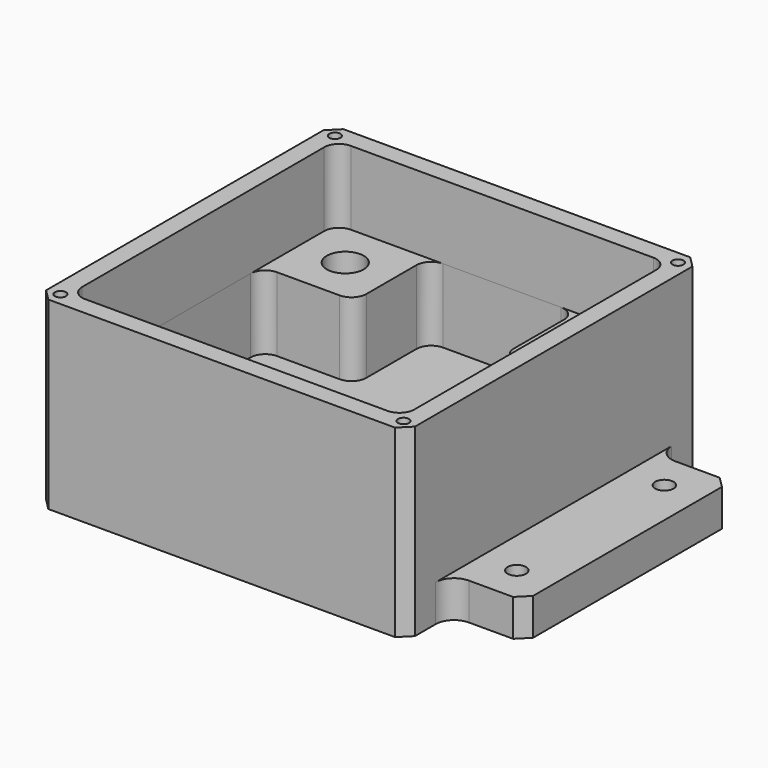
from build123d import *

# Parameters (mm, degrees)
F1_DEPTH     = 50
F2_W         = 20
F2_H         = 100
F3_DEPTH     = 40
F4_R         = 2.5
F5_DEPTH     = 10
F6_W         = 90
F6_H         = 90
F7_DEPTH     = 20
F8_R         = 5
F9_DEPTH     = 20
F10_R        = 1.5
F11_DEPTH    = 40
F12_SIZE     = 3
F13_T1_DEPTH = 30
F13_T3_DEPTH = 30
F13_T5_DEPTH = 30


# Not quite as in the source:
# - a fillet or chamfer that OpenCascade refuses, or shapes differently, is made with other operations: its cross-section is extruded or revolved along the edge and cut away or added


with BuildPart() as f1:
    # F0 (on Top) → F1 (new body)
    with BuildSketch(Plane.XY):
        Polygon((-50, -50), (50, -50), (70, -50), (70, 50), (50, 50), (-50, 50), align=None)
    extrude(amount=F1_DEPTH)

    # F2 (on face) → F3 (cut)
    with BuildSketch(Plane.XY.offset(50)):
        with Locations((60, 0)):
            Rectangle(F2_W, F2_H)
    extrude(amount=-F3_DEPTH, mode=Mode.SUBTRACT)

    # F4 (on face) → F5 (cut, through all)
    with BuildSketch(Plane.XY.offset(10)):
        with BuildLine():
            Line((50, -40), (50, -50))
            Line((50, -50), (70, -50))
            Line((70, -50), (70, -35))
            Line((70, -35), (55, -35))
            ThreePointArc((55, -35), (51.4644660941, -36.4644660941), (50, -40))
        make_face()
        with Locations((60, -25)):
            Circle(F4_R)
        with Locations((60, 25)):
            Circle(F4_R)
        with BuildLine():
            ThreePointArc((50, 40), (51.4644660941, 36.4644660941), (55, 35))
            Line((55, 35), (70, 35))
            Line((70, 35), (70, 50))
            Line((70, 50), (50, 50))
            Line((50, 50), (50, 40))
        make_face()
    extrude(amount=-F5_DEPTH, mode=Mode.SUBTRACT)

    # F6 (on face) → F7 (cut)
    with BuildSketch(Plane.XY.offset(50)):
        Rectangle(F6_W, F6_H)
    extrude(amount=-F7_DEPTH, mode=Mode.SUBTRACT)

    # F8 (on face) → F9 (cut)
    with BuildSketch(Plane.XY.offset(30)):
        with Locations((-32.5000025332, 32.5000174344)):
            Circle(F8_R)
        Polygon((-45.0000017881, 20.0000017881), (-45.0000017881, -20.0000017881), (-20.0000017881, -20.0000017881), (-20.0000017881, -45.0000017881), (20.0000017881, -45.0000017881), (20.0000017881, -20.0000017881), (45.0000017881, -20.0000017881), (45.0000017881, 20.0000017881), (20.0000017881, 20.0000017881), (20.0000017881, 45.0000017881), (-20.0000017881, 45.0000017881), (-20.0000017881, 20.0000017881), align=None)
        with Locations((-32.5000025332, -32.5000174344)):
            Circle(F8_R)
        with Locations((32.5000025332, 32.5000174344)):
            Circle(F8_R)
        with Locations((32.5000025332, -32.5000174344)):
            Circle(F8_R)
    extrude(amount=-F9_DEPTH, mode=Mode.SUBTRACT)

    # F10 (on face) → F11 (cut)
    with BuildSketch(Plane.XY.offset(50)):
        with Locations((-46.5, 46.5)):
            Circle(F10_R)
        with Locations((-46.5, -46.5)):
            Circle(F10_R)
        with Locations((46.5, 46.5)):
            Circle(F10_R)
        with Locations((46.5, -46.5)):
            Circle(F10_R)
    extrude(amount=-F11_DEPTH, mode=Mode.SUBTRACT)

    # F12
    f12_edges = [f1.edges().sort_by_distance(p)[0] for p in [
        (70, -35, 5),
        (70, 35, 5),
        (50, -50, 25),
        (-50, -50, 25),
        (50, 50, 25),
        (-50, 50, 25),
    ]]
    chamfer(f12_edges, length=F12_SIZE)

    # F13: fillet of radius 4 on 16 edges, made by hand

    # F13_s2 → F13_t1 (join)
    with BuildSketch(Plane.XY.offset(20)):
        with BuildLine():
            ThreePointArc((-45, 41), (-43.8284271247, 43.8284271247), (-41, 45))
            Line((-41, 45), (-45, 45))
            Line((-45, 45), (-45, 41))
        make_face()
        with BuildLine():
            ThreePointArc((45, 41), (43.8284271247, 43.8284271247), (41, 45))
            Line((41, 45), (45, 45))
            Line((45, 45), (45, 41))
        make_face()
        with BuildLine():
            ThreePointArc((41, -45), (43.8284271247, -43.8284271247), (45, -41))
            Line((45, -41), (45, -45))
            Line((45, -45), (41, -45))
        make_face()
        with BuildLine():
            ThreePointArc((-41, -45), (-43.8284271247, -43.8284271247), (-45, -41))
            Line((-45, -41), (-45, -45))
            Line((-45, -45), (-41, -45))
        make_face()
    extrude(amount=F13_T1_DEPTH)

    # F13_s4 → F13_t3 (join)
    with BuildSketch(Plane.XY):
        with BuildLine():
            ThreePointArc((-41.0000017881, 20.0000017881), (-43.8284289129, 18.8284289129), (-45.0000017881, 16.0000017881))
            Line((-45.0000017881, 16.0000017881), (-45.0000017881, 20.0000017881))
            Line((-45.0000017881, 20.0000017881), (-41.0000017881, 20.0000017881))
        make_face()
        with BuildLine():
            ThreePointArc((-20.0000017881, 41.0000017881), (-18.8284289129, 43.8284289129), (-16.0000017881, 45.0000017881))
            Line((-16.0000017881, 45.0000017881), (-20.0000017881, 45.0000017881))
            Line((-20.0000017881, 45.0000017881), (-20.0000017881, 41.0000017881))
        make_face()
        with BuildLine():
            ThreePointArc((20.0000017881, 41.0000017881), (18.8284289129, 43.8284289129), (16.0000017881, 45.0000017881))
            Line((16.0000017881, 45.0000017881), (20.0000017881, 45.0000017881))
            Line((20.0000017881, 45.0000017881), (20.0000017881, 41.0000017881))
        make_face()
        with BuildLine():
            ThreePointArc((41.0000017881, 20.0000017881), (43.8284289129, 18.8284289129), (45.0000017881, 16.0000017881))
            Line((45.0000017881, 16.0000017881), (45.0000017881, 20.0000017881))
            Line((45.0000017881, 20.0000017881), (41.0000017881, 20.0000017881))
        make_face()
        with BuildLine():
            ThreePointArc((-41.0000017881, -20.0000017881), (-43.8284289129, -18.8284289129), (-45.0000017881, -16.0000017881))
            Line((-45.0000017881, -16.0000017881), (-45.0000017881, -20.0000017881))
            Line((-45.0000017881, -20.0000017881), (-41.0000017881, -20.0000017881))
        make_face()
        with BuildLine():
            ThreePointArc((-20.0000017881, -41.0000017881), (-18.8284289129, -43.8284289129), (-16.0000017881, -45.0000017881))
            Line((-16.0000017881, -45.0000017881), (-20.0000017881, -45.0000017881))
            Line((-20.0000017881, -45.0000017881), (-20.0000017881, -41.0000017881))
        make_face()
        with BuildLine():
            ThreePointArc((20.0000017881, -41.0000017881), (18.8284289129, -43.8284289129), (16.0000017881, -45.0000017881))
            Line((16.0000017881, -45.0000017881), (20.0000017881, -45.0000017881))
            Line((20.0000017881, -45.0000017881), (20.0000017881, -41.0000017881))
        make_face()
        with BuildLine():
            ThreePointArc((41.0000017881, -20.0000017881), (43.8284289129, -18.8284289129), (45.0000017881, -16.0000017881))
            Line((45.0000017881, -16.0000017881), (45.0000017881, -20.0000017881))
            Line((45.0000017881, -20.0000017881), (41.0000017881, -20.0000017881))
        make_face()
    extrude(amount=F13_T3_DEPTH)

    # F13_s6 → F13_t5 (cut)
    with BuildSketch(Plane.XY.offset(10)):
        with BuildLine():
            ThreePointArc((-20.0000017881, 24.0000017881), (-21.1715746634, 21.1715746634), (-24.0000017881, 20.0000017881))
            Line((-24.0000017881, 20.0000017881), (-20.0000017881, 20.0000017881))
            Line((-20.0000017881, 20.0000017881), (-20.0000017881, 24.0000017881))
        make_face()
        with BuildLine():
            ThreePointArc((24.0000017881, 20.0000017881), (21.1715746634, 21.1715746634), (20.0000017881, 24.0000017881))
            Line((20.0000017881, 24.0000017881), (20.0000017881, 20.0000017881))
            Line((20.0000017881, 20.0000017881), (24.0000017881, 20.0000017881))
        make_face()
        with BuildLine():
            ThreePointArc((-24.0000017881, -20.0000017881), (-21.1715746634, -21.1715746634), (-20.0000017881, -24.0000017881))
            Line((-20.0000017881, -24.0000017881), (-20.0000017881, -20.0000017881))
            Line((-20.0000017881, -20.0000017881), (-24.0000017881, -20.0000017881))
        make_face()
        with BuildLine():
            ThreePointArc((24.0000017881, -20.0000017881), (21.1715746634, -21.1715746634), (20.0000017881, -24.0000017881))
            Line((20.0000017881, -24.0000017881), (20.0000017881, -20.0000017881))
            Line((20.0000017881, -20.0000017881), (24.0000017881, -20.0000017881))
        make_face()
    extrude(amount=F13_T5_DEPTH, mode=Mode.SUBTRACT)


solid = f1.part
